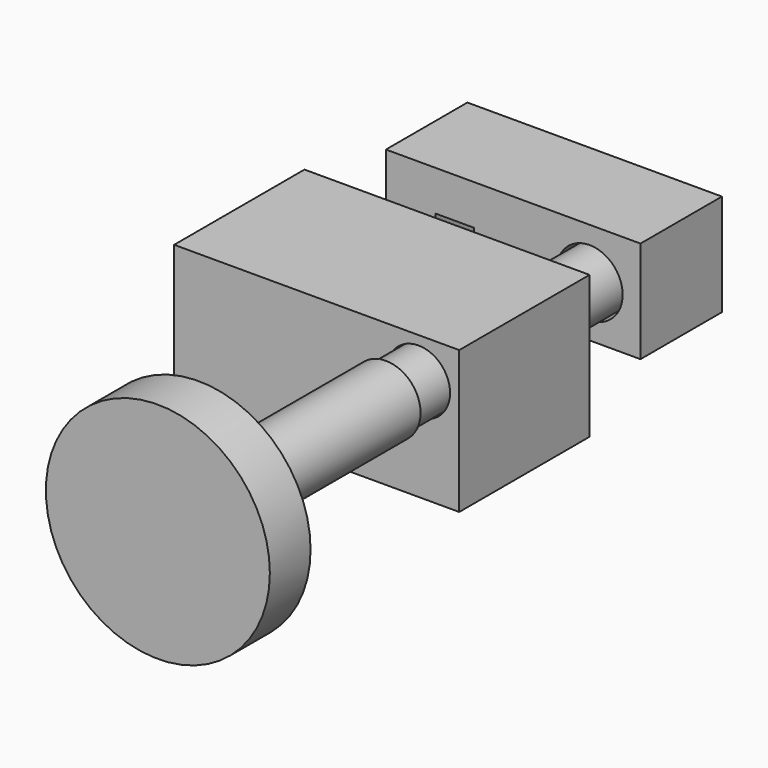
from build123d import *

# Parameters (mm, degrees)
F0_W      = 28
F0_H      = 4.3
F0_H_2    = 9.7
F0_W_2    = 13.5
F0_H_3    = 7.7
F0_R      = 3.1
F1_DEPTH  = 16
F2_W      = 13.5
F2_H      = 7.7
F3_DEPTH  = 2
F4_R      = 1.1
F5_DEPTH  = 12
F8_R      = 11
F9_DEPTH  = 5
F10_R     = 3
F11_DEPTH = 48
F12_W     = 25
F12_H     = 10
F13_DEPTH = 10
F14_W     = 3.8
F14_H     = 3.8
F15_DEPTH = 7
F14_R     = 3.25
F16_DEPTH = 8.5
F17_R     = 3.4
F18_DEPTH = 23
F19_R     = 3
F20_DEPTH = 7.5
F21_R     = 1.1
F22_DEPTH = 12
F23_R     = 1.6
F24_DEPTH = 25


with BuildPart() as f1:
    # F0 (on Front) → F1 (new body)
    with BuildSketch(Plane.XZ):
        with Locations((-36, -7)):
            Rectangle(F0_W, F0_H)
        with Locations((-36, 0)):
            Rectangle(F0_W, F0_H_2)
        with Locations((-41.75, 0)):
            Rectangle(F0_W_2, F0_H_3, mode=Mode.SUBTRACT)
        with Locations((-26, 0.85)):
            Circle(F0_R, mode=Mode.SUBTRACT)
    extrude(amount=-F1_DEPTH)

    # F2 (on face) → F3 (join)
    with BuildSketch(Plane.XZ):
        with Locations((-41.75, 0)):
            Rectangle(F2_W, F2_H)
    extrude(amount=-F3_DEPTH)

    # F4 (on face) → F5 (cut)
    with BuildSketch(Plane(origin=(0, 0, -9.15), x_dir=(1, 0, 0), z_dir=(0, 0, -1))):
        with Locations((-32, -3.5)):
            Circle(F4_R)
        with Locations((-32, -12.5)):
            Circle(F4_R)
    extrude(amount=-F5_DEPTH, mode=Mode.SUBTRACT)


with BuildPart() as f9:
    # F8 (on offset) → F9 (new body)
    with BuildSketch(Plane.XZ.offset(27)):
        with Locations((-26, 0.85)):
            Circle(F8_R)
    extrude(amount=F9_DEPTH)

    # F10 (on face) → F11 (join)
    with BuildSketch(Plane(origin=(0, -27, 0), x_dir=(-1, 0, 0), z_dir=(0, 1, 0))):
        with Locations((26, 0.85)):
            Circle(F10_R)
    extrude(amount=F11_DEPTH)

    # F17 (on face) → F18 (join)
    with BuildSketch(Plane.XZ.offset(27)):
        with Locations((-26, 0.85)):
            Circle(F17_R)
    extrude(amount=-F18_DEPTH)

    # F19 (on face) → F20 (join)
    with BuildSketch(Plane(origin=(0, 21, 0), x_dir=(-1, 0, 0), z_dir=(0, 1, 0))):
        with Locations((26, 0.85)):
            Circle(F19_R)
    extrude(amount=F20_DEPTH)

    # F21 (on face) → F22 (cut)
    with BuildSketch(Plane(origin=(0, 28.5, 0), x_dir=(-1, 0, 0), z_dir=(0, 1, 0))):
        with Locations((26, 0.85)):
            Circle(F21_R)
    extrude(amount=-F22_DEPTH, mode=Mode.SUBTRACT)


with BuildPart() as f13:
    # F12 (on offset) → F13 (new body)
    with BuildSketch(Plane(origin=(0, 21, 0), x_dir=(-1, 0, 0), z_dir=(0, 1, 0))):
        with Locations((33.5, 0.85)):
            Rectangle(F12_W, F12_H)
    extrude(amount=F13_DEPTH)

    # F14 (on face) → F15 (cut)
    with BuildSketch(Plane.XZ.offset(-21)):
        with Locations((-39.25, 0)):
            Rectangle(F14_W, F14_H)
    extrude(amount=-F15_DEPTH, mode=Mode.SUBTRACT)

    # F14 (on face) → F16 (cut)
    with BuildSketch(Plane.XZ.offset(-21)):
        with Locations((-26, 0.85)):
            Circle(F14_R)
    extrude(amount=-F16_DEPTH, mode=Mode.SUBTRACT)

    # F23 (on face) → F24 (cut)
    with BuildSketch(Plane(origin=(0, 31, 0), x_dir=(-1, 0, 0), z_dir=(0, 1, 0))):
        with Locations((26, 0.85)):
            Circle(F23_R)
    extrude(amount=-F24_DEPTH, mode=Mode.SUBTRACT)


solid = Compound([f1.part, f9.part, f13.part])
